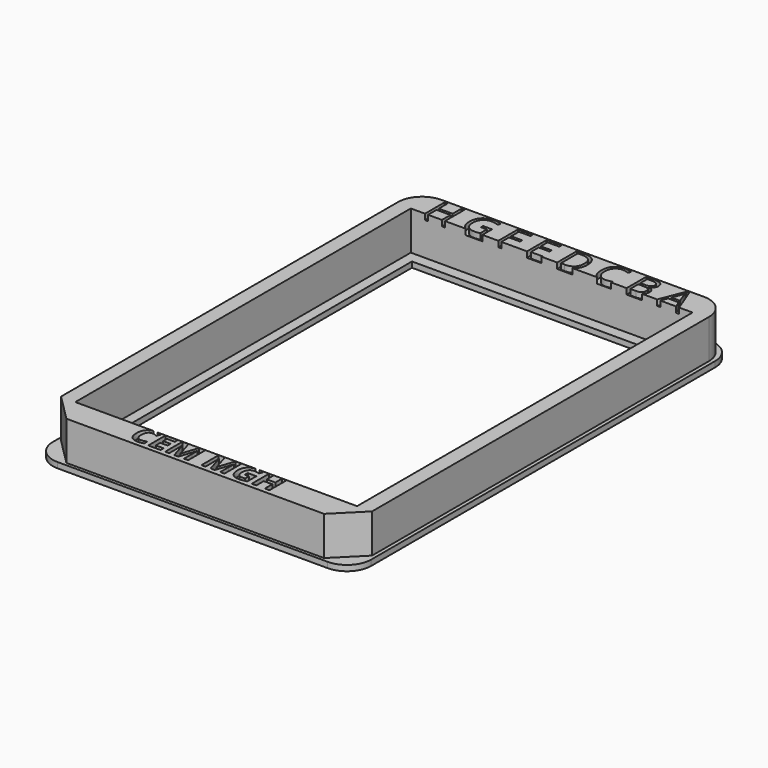
from build123d import *

# Parameters (mm, degrees)
F1_DEPTH       = 11.7
F2_W           = 68.834
F2_H           = 104.4194
F3_DEPTH       = 18.542
F4_W           = 74.0664
F4_H           = 110.236
F4_W_2         = 68.834
F4_H_2         = 104.4194
F5_DEPTH       = 10.22858
F6_TEXT_SIZE   = 9.7107964115
F6_TEXT_SIZE_2 = 7.9375
F7_DEPTH       = 1.5


# Not quite as in the source:
# - a feature names something its author has since deleted; it is built from what else it names
# - Text() gives the source's letters only with a copy of the font that has no kerning and outlines rounded to 1/6400 em; it was checked with that copy


with BuildPart() as f1:
    # F0 (on Top) → F1 (new body)
    with BuildSketch(Plane.XY):
        with BuildLine():
            Line((35.4965, 62.865), (-35.4965, 62.865))
            ThreePointArc((-35.4965, 62.865), (-39.9866280605, 61.0051280605), (-41.8465, 56.515))
            Line((-41.8465, 56.515), (-41.8465, -56.515))
            ThreePointArc((-41.8465, -56.515), (-39.9866280605, -61.0051280605), (-35.4965, -62.865))
            Line((-35.4965, -62.865), (35.4965, -62.865))
            ThreePointArc((35.4965, -62.865), (39.9866280605, -61.0051280605), (41.8465, -56.515))
            Line((41.8465, -56.515), (41.8465, 56.515))
            ThreePointArc((41.8465, 56.515), (39.9866280605, 61.0051280605), (35.4965, 62.865))
        make_face()
    extrude(amount=F1_DEPTH)

    # F2 (on face) → F3 (cut)
    with BuildSketch(Plane.XY.offset(11.7)):
        Rectangle(F2_W, F2_H)
    extrude(amount=-F3_DEPTH, mode=Mode.SUBTRACT)

    # F4 (on face) → F5 (cut)
    with BuildSketch(Plane.XY.offset(11.7)):
        with BuildLine():
            ThreePointArc((41.8465, 56.515), (39.9866280605, 61.0051280605), (35.4965, 62.865))
            Line((35.4965, 62.865), (-35.4965, 62.865))
            ThreePointArc((-35.4965, 62.865), (-39.9866280605, 61.0051280605), (-41.8465, 56.515))
            Line((-41.8465, 56.515), (-41.8465, -56.515))
            ThreePointArc((-41.8465, -56.515), (-39.9866280605, -61.0051280605), (-35.4965, -62.865))
            Line((-35.4965, -62.865), (35.4965, -62.865))
            ThreePointArc((35.4965, -62.865), (39.9866280605, -61.0051280605), (41.8465, -56.515))
            Line((41.8465, -56.515), (41.8465, 56.515))
        make_face()
        with BuildLine():
            ThreePointArc((-40.87495, 55.68315), (-39.0150780605, 60.1732780605), (-34.52495, 62.03315))
            Line((-34.52495, 62.03315), (34.52495, 62.03315))
            ThreePointArc((34.52495, 62.03315), (39.0150780605, 60.1732780605), (40.87495, 55.68315))
            Line((40.87495, 55.68315), (40.87495, -55.02275))
            Line((40.87495, -55.02275), (33.86455, -62.03315))
            Line((33.86455, -62.03315), (-33.86455, -62.03315))
            Line((-33.86455, -62.03315), (-40.87495, -55.02275))
            Line((-40.87495, -55.02275), (-40.87495, 55.68315))
        make_face(mode=Mode.SUBTRACT)
        with Locations((-0.0127, 0)):
            Rectangle(F4_W, F4_H)
        Rectangle(F4_W_2, F4_H_2, mode=Mode.SUBTRACT)
    extrude(amount=-F5_DEPTH, mode=Mode.SUBTRACT)

    # F6 (on face) → F7 (cut)
    with BuildSketch(Plane.XY.offset(11.7)):
        with Locations((-34.2742875249, 54.6603765837)):
            Text('H G F E D C B A', F6_TEXT_SIZE, font='Open Sans', text_align=(TextAlign.LEFT, TextAlign.BOTTOM))
        with Locations((-19.0881248047, -60.833)):
            Text('CEM MGH', F6_TEXT_SIZE_2, font='Open Sans', font_style=FontStyle.BOLD, text_align=(TextAlign.LEFT, TextAlign.BOTTOM))
    extrude(amount=-F7_DEPTH, mode=Mode.SUBTRACT)


solid = f1.part
